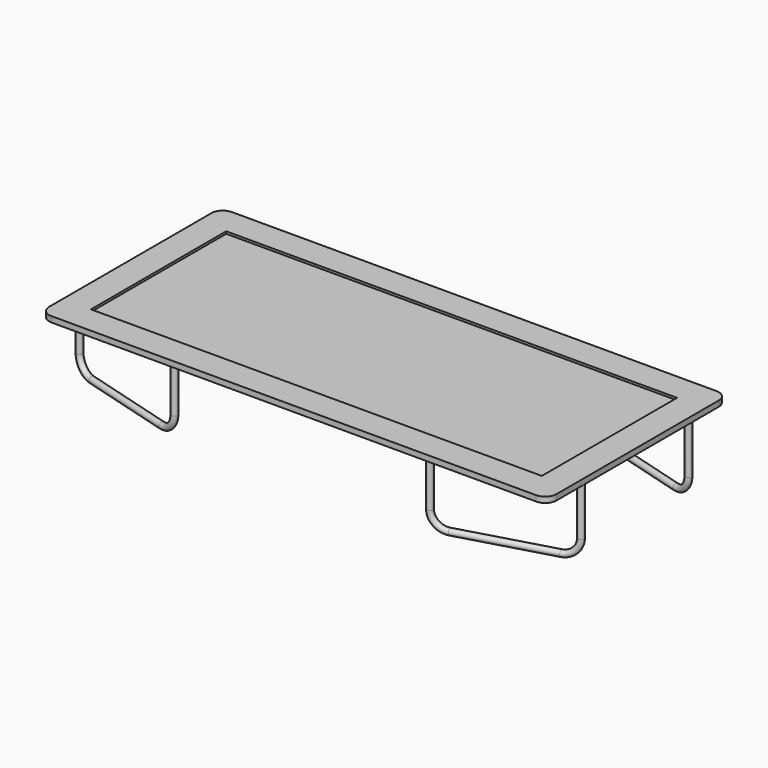
from build123d import *

# Parameters (mm, degrees)
F0_W              = 4500
F0_H              = 2000
F1_DEPTH          = 50
F2_W              = 4000
F2_H              = 1500
F3_DEPTH          = 20
F4_R              = 100
F9_R              = 27.6060053196
F10_COPIES2_COUNT = 2


# Not quite as in the source:
# - a feature of the source that left no trace in its solid (it failed there, or was rolled back) is left out
# - a pattern or mirror of a feature is missing from the dataset's text; its kind, count and spacing are read off the source's solid


with BuildPart() as f1:
    # F0 (on Top) → F1 (new body)
    with BuildSketch(Plane.XY):
        Rectangle(F0_W, F0_H)
    extrude(amount=F1_DEPTH)

    # F2 (on face) → F3 (cut)
    with BuildSketch(Plane.XY.offset(50)):
        Rectangle(F2_W, F2_H)
    extrude(amount=-F3_DEPTH, mode=Mode.SUBTRACT)

    # F4
    f4_edges = [f1.edges().sort_by_distance(p)[0] for p in [
        (-2250, -1000, 25),
        (2250, -1000, 25),
        (2250, 1000, 25),
        (-2250, 1000, 25),
    ]]
    fillet(f4_edges, radius=F4_R)

    # F10: sweep along a path in F8
    with BuildLine(Plane(origin=(-301.8867924528, -1056.6037735849, 0), x_dir=(-0.9615239476, 0.2747211279, 0), z_dir=(0.2747211279, 0.9615239476, 0))) as f10_path:
        Line((2026.0683182432, 0), (2026.0683182432, -423.2082843781))
        ThreePointArc((2026.0683182432, -423.2082843781), (1967.4896744805, -564.6296406154), (1826.0683182432, -623.2082843781))
        Line((1826.0683182432, -623.2082843781), (989.750339326, -623.2082843781))
        ThreePointArc((989.750339326, -623.2082843781), (848.4542193127, -564.754766034), (789.7506527308, -423.5623490699))
        Line((789.7506527308, -423.5623490699), (789.0008091927, 0))
    # F9 (on face) → F10 (sweep)
    with BuildSketch(Plane.XY):
        with Locations((-2224.6488836829, -595.6394452545)):
            Circle(F9_R)
    f10 = sweep(path=f10_path.line)

    # F10_copies: F10 across plane
    add(f10.mirror(Plane.ZX))

    # F10_copies1: F10 across plane
    add(f10.mirror(Plane(origin=(0, 0, 0), x_dir=(0, 0, 1), z_dir=(1, 0, 0))))

    # F10_copies2: F10 ×2 about axis
    f10_copies2_axis = Axis((0, 0, 0), (0, 0, 1))
    for i in range(1, F10_COPIES2_COUNT):
        add(f10.rotate(f10_copies2_axis, i * 360 / F10_COPIES2_COUNT))


solid = f1.part
